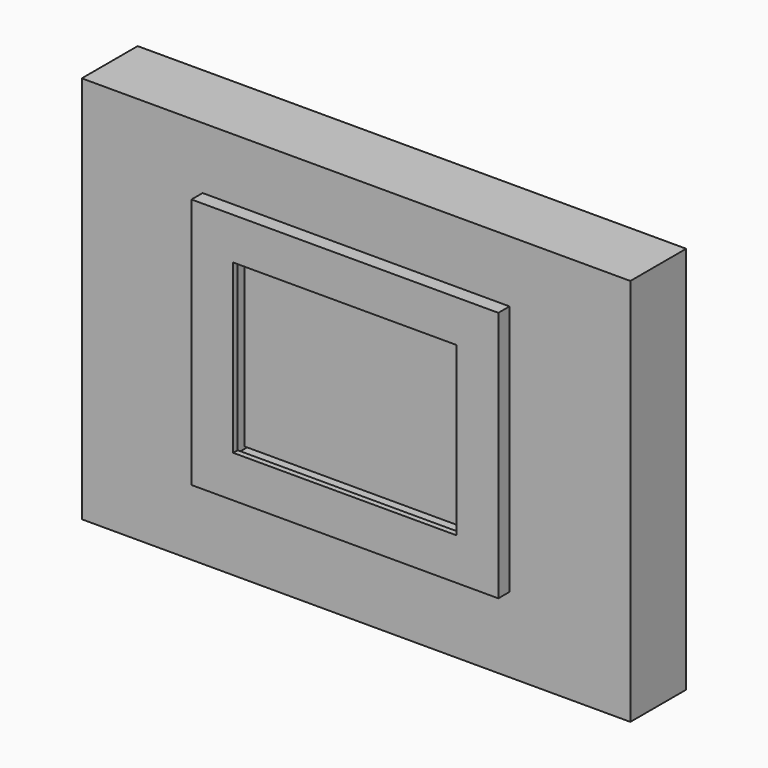
from build123d import *

# Parameters (mm, degrees)
F0_W         = 80
F0_H         = 60
F1_DEPTH     = 25
F2_W         = 196.4207142591
F2_H         = 138.9969103038
F2_W_2       = 90
F2_H_2       = 70
F3_DEPTH     = 25
F4_W         = 109.8849922419
F4_H         = 90
F4_W_2       = 80
F4_H_2       = 60
F5_DEPTH     = 5
F6_T1_DEPTH  = 80
F6_T3_DEPTH  = 60
F6_T9_DEPTH  = 67.7150489639
F6_T14_DEPTH = 87.7150489639
F6_T22_DEPTH = 87.7150489639
F6_T27_DEPTH = 67.7150489639
F6_T35_DEPTH = 87.7150489639
F6_T40_DEPTH = 67.7150489639
F6_T48_DEPTH = 67.7150489639
F6_T53_DEPTH = 87.7150489639


# Not quite as in the source:
# - a fillet or chamfer that OpenCascade refuses, or shapes differently, is made with other operations: its cross-section is extruded or revolved along the edge and cut away or added


with BuildPart() as f1:
    # F0 (on Front) → F1 (new body)
    with BuildSketch(Plane.XZ):
        Rectangle(F0_W, F0_H)
    extrude(amount=-F1_DEPTH)



with BuildPart() as f3:
    # F2 (on face) → F3 (new body)
    with BuildSketch(Plane.XZ):
        with Locations((0, -2.4136770517)):
            Rectangle(F2_W, F2_H)
        Rectangle(F2_W_2, F2_H_2, mode=Mode.SUBTRACT)
    extrude(amount=-F3_DEPTH)


with BuildPart() as f1_1:
    add(f1.part)

    add(f3.part)  # F5 merges F3
    # F4 (on face) → F5 (join)
    with BuildSketch(Plane.XZ):
        Rectangle(F4_W, F4_H)
        Rectangle(F4_W_2, F4_H_2, mode=Mode.SUBTRACT)
    extrude(amount=F5_DEPTH)

    # F6: chamfer of 3 on 4 edges, made by hand

    # F6_s2 → F6_t1 (cut)
    with BuildSketch(Plane.YZ.offset(-40)):
        Polygon((0, 33), (-3, 30), (0, 30), align=None)
        Polygon((0, -33), (-3, -30), (0, -30), align=None)
    extrude(amount=F6_T1_DEPTH, mode=Mode.SUBTRACT)

    # F6_s4 → F6_t3 (cut)
    with BuildSketch(Plane.XY.offset(-30)):
        Polygon((-43, 0), (-40, -3), (-40, 0), align=None)
        Polygon((43, 0), (40, -3), (40, 0), align=None)
    extrude(amount=F6_T3_DEPTH, mode=Mode.SUBTRACT)


with BuildPart() as f6_tool7:
    # F6_s8 → F6_t9 (new body)
    with BuildSketch(Plane.XY.offset(-30)):
        Polygon((43, 0), (40, -3), (40, 0), align=None)
    extrude(amount=F6_T9_DEPTH)

    split(bisect_by=Plane.XY.offset(35), keep=Keep.BOTTOM)

    split(bisect_by=Plane.XY.offset(30), keep=Keep.TOP)


with BuildPart() as f6_tool12:
    # F6_s13 → F6_t14 (new body)
    with BuildSketch(Plane.YZ.offset(47.7150489639)):
        Polygon((0, 33), (-3, 30), (0, 30), align=None)
    extrude(amount=-F6_T14_DEPTH)

    split(bisect_by=Plane.YZ.offset(45), keep=Keep.BOTTOM)

    split(bisect_by=Plane.YZ.offset(40), keep=Keep.TOP)


with BuildPart() as f6_tool7_1:
    add(f6_tool7.part)

    # F6_t17: intersect F6_tool12
    add(f6_tool12.part, mode=Mode.INTERSECT)


with BuildPart() as f1_2:
    add(f1_1.part)

    # F6_t5: cut F6_tool7
    add(f6_tool7_1.part, mode=Mode.SUBTRACT)


with BuildPart() as f6_tool20:
    # F6_s21 → F6_t22 (new body)
    with BuildSketch(Plane.YZ.offset(40)):
        Polygon((0, 33), (-3, 30), (0, 30), align=None)
    extrude(amount=-F6_T22_DEPTH)

    split(bisect_by=Plane.YZ.offset(-45), keep=Keep.TOP)

    split(bisect_by=Plane.YZ.offset(-40), keep=Keep.BOTTOM)


with BuildPart() as f6_tool25:
    # F6_s26 → F6_t27 (new body)
    with BuildSketch(Plane.XY.offset(37.7150489639)):
        Polygon((-43, 0), (-40, -3), (-40, 0), align=None)
    extrude(amount=-F6_T27_DEPTH)

    split(bisect_by=Plane.XY.offset(35), keep=Keep.BOTTOM)

    split(bisect_by=Plane.XY.offset(30), keep=Keep.TOP)


with BuildPart() as f6_tool20_1:
    add(f6_tool20.part)

    # F6_t30: intersect F6_tool25
    add(f6_tool25.part, mode=Mode.INTERSECT)


with BuildPart() as f1_3:
    add(f1_2.part)

    # F6_t18: cut F6_tool20
    add(f6_tool20_1.part, mode=Mode.SUBTRACT)


with BuildPart() as f6_tool33:
    # F6_s34 → F6_t35 (new body)
    with BuildSketch(Plane.YZ.offset(-47.7150489639)):
        Polygon((0, -33), (-3, -30), (0, -30), align=None)
    extrude(amount=F6_T35_DEPTH)

    split(bisect_by=Plane.YZ.offset(-45), keep=Keep.TOP)

    split(bisect_by=Plane.YZ.offset(-40), keep=Keep.BOTTOM)


with BuildPart() as f6_tool38:
    # F6_s39 → F6_t40 (new body)
    with BuildSketch(Plane.XY.offset(30)):
        Polygon((-43, 0), (-40, -3), (-40, 0), align=None)
    extrude(amount=-F6_T40_DEPTH)

    split(bisect_by=Plane.XY.offset(-35), keep=Keep.TOP)

    split(bisect_by=Plane.XY.offset(-30), keep=Keep.BOTTOM)


with BuildPart() as f6_tool33_1:
    add(f6_tool33.part)

    # F6_t43: intersect F6_tool38
    add(f6_tool38.part, mode=Mode.INTERSECT)


with BuildPart() as f1_4:
    add(f1_3.part)

    # F6_t31: cut F6_tool33
    add(f6_tool33_1.part, mode=Mode.SUBTRACT)


with BuildPart() as f6_tool46:
    # F6_s47 → F6_t48 (new body)
    with BuildSketch(Plane.XY.offset(-37.7150489639)):
        Polygon((43, 0), (40, -3), (40, 0), align=None)
    extrude(amount=F6_T48_DEPTH)

    split(bisect_by=Plane.XY.offset(-35), keep=Keep.TOP)

    split(bisect_by=Plane.XY.offset(-30), keep=Keep.BOTTOM)


with BuildPart() as f6_tool51:
    # F6_s52 → F6_t53 (new body)
    with BuildSketch(Plane.YZ.offset(-40)):
        Polygon((0, -33), (-3, -30), (0, -30), align=None)
    extrude(amount=F6_T53_DEPTH)

    split(bisect_by=Plane.YZ.offset(45), keep=Keep.BOTTOM)

    split(bisect_by=Plane.YZ.offset(40), keep=Keep.TOP)


with BuildPart() as f6_tool46_1:
    add(f6_tool46.part)

    # F6_t56: intersect F6_tool51
    add(f6_tool51.part, mode=Mode.INTERSECT)


with BuildPart() as f1_5:
    add(f1_4.part)

    # F6_t44: cut F6_tool46
    add(f6_tool46_1.part, mode=Mode.SUBTRACT)


solid = f1_5.part
